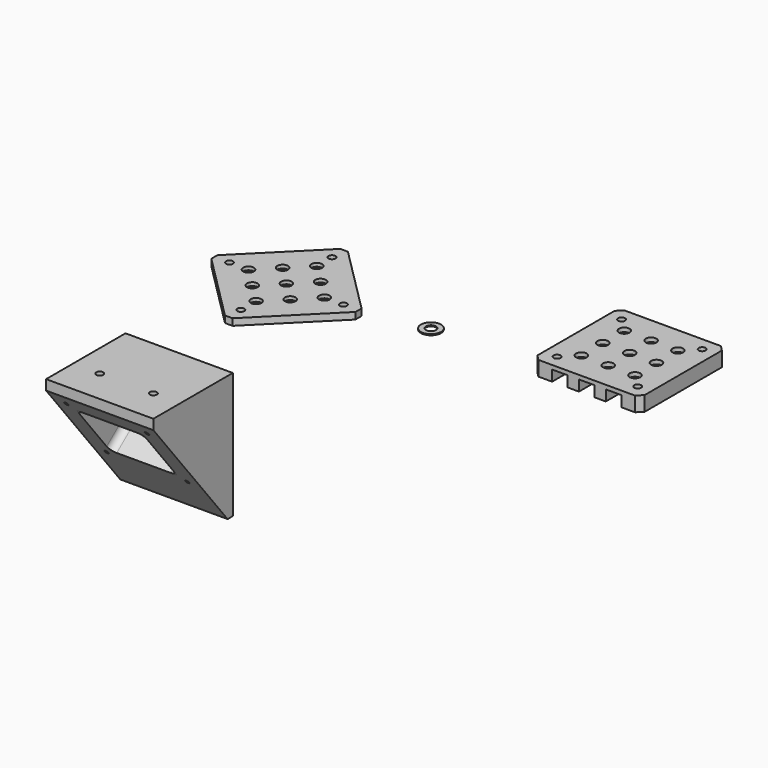
from build123d import *
from build123d import SkipClean  # not in build123d's __all__

# Parameters (mm, degrees)
F1_DEPTH        = 6.35
F2_D            = 6.604
F4_D            = 10.0838
F4_CBORE_D      = 19.558
F4_CBORE_DEPTH  = 3.175
F5_SIZE         = 5.08
F6_W            = 101.6
F6_H            = 101.6
F7_DEPTH        = 13.97
F9_D            = 6.604
F10_W           = 14.732
F10_H           = 10.16
F11_DEPTH       = 101.601
F12_SIZE        = 5.08
F13_R           = 9.525
F13_R_2         = 4.7625
F14_DEPTH       = 1.016
F16_DEPTH       = 50.8
F18_D           = 3.96875
F18_DEPTH       = 12.7
F18_TIP         = 1.1923327909
F20_DEPTH       = 119.0509465201
F22_D           = 6.604
F22_CBORE_D     = 10.16
F22_CBORE_DEPTH = 114.3
F23_W           = 63.5
F23_H           = 63.5
F24_DEPTH       = 31.75
F26_D           = 10.0838
F26_DEPTH       = 25.4
F26_TIP         = 3.0294791551
F27_T1_DEPTH    = 47.625
F27_T6_DEPTH    = 31.75
F27_S7_R        = 5.08
F27_T8_DEPTH    = 21
F27_T12_DEPTH   = 31.75
F27_S13_R       = 5.08
F27_T14_DEPTH   = 21


# Not quite as in the source:
# - a fillet or chamfer that OpenCascade refuses, or shapes differently, is made with other operations: its cross-section is extruded or revolved along the edge and cut away or added


with BuildPart() as f1:
    # F0 (on Top) → F1 (new body)
    with BuildSketch(Plane.XY):
        Polygon((-71.8420489686, 0), (0, -71.8420489686), (71.8420489686, 0), (0, 71.8420489686), align=None)
    extrude(amount=F1_DEPTH)

    # F2 (through all)
    with Locations(Plane(origin=(0, 0, 0), x_dir=(1, 0, 0), z_dir=(0, 0, -1))):
        with Locations((0, 53.975), (-53.975, 0), (53.975, 0), (0, -53.975)):
            Hole(F2_D / 2)

    # F4 (through all)
    with Locations(Plane(origin=(0, 0, 0), x_dir=(1, 0, 0), z_dir=(0, 0, -1))):
        with Locations((0, 35.9210244843), (-17.9605122421, 17.9605122421), (-35.9210244843, 0), (-17.9605122421, -17.9605122421), (0, -35.9210244843), (17.9605122421, -17.9605122421), (35.9210244843, 0), (17.9605122421, 17.9605122421), (0, 0)):
            CounterBoreHole(F4_D / 2, F4_CBORE_D / 2, F4_CBORE_DEPTH)

    # F5
    f5_edges = [f1.edges().sort_by_distance(p)[0] for p in [
        (-71.842049, 0, 3.175),
        (0, 71.842049, 3.175),
        (71.842049, 0, 3.175),
        (0, -71.842049, 3.175),
    ]]
    chamfer(f5_edges, length=F5_SIZE)


with BuildPart() as f7:
    # F6 (on face) → F7 (new body)
    with BuildSketch(Plane.XY.offset(6.35)):
        with Locations((284.3260511961, 50.8)):
            Rectangle(F6_W, F6_H)
    extrude(amount=F7_DEPTH)

    # F9 (through all)
    with Locations(Plane(origin=(0, 0, 6.35), x_dir=(1, 0, 0), z_dir=(0, 0, -1))):
        with Locations((246.1599626816, -88.9660885145), (246.1599626816, -12.6339114855), (322.4921397107, -12.6339114855), (322.4921397107, -88.9660885145)):
            Hole(F9_D / 2)

    # F10 (on face) → F11 (cut, through all)
    with BuildSketch(Plane.XZ):
        with Locations((309.7260511961, 11.43)):
            Rectangle(F10_W, F10_H)
        with Locations((284.3260511961, 11.43)):
            Rectangle(F10_W, F10_H)
        with Locations((258.9260511961, 11.43)):
            Rectangle(F10_W, F10_H)
    extrude(amount=-F11_DEPTH, mode=Mode.SUBTRACT)

    # F12
    f12_edges = [f7.edges().sort_by_distance(p)[0] for p in [
        (335.126051, 0, 13.335),
        (233.526051, 0, 13.335),
        (233.526051, 101.6, 13.335),
        (335.126051, 101.6, 13.335),
    ]]
    chamfer(f12_edges, length=F12_SIZE)

    # F26
    with Locations(Plane(origin=(0, 0, 16.51), x_dir=(1, 0, 0), z_dir=(0, 0, -1))):
        with Locations((258.9260511961, -25.4), (258.9260511961, -50.8), (258.9260511961, -76.2), (284.3260511961, -76.2), (284.3260511961, -50.8), (284.3260511961, -25.4), (309.7260511961, -25.4), (309.7260511961, -50.8), (309.7260511961, -76.2)):
            Hole(F26_D / 2, depth=F26_DEPTH)
            with Locations((0, 0, -(F26_DEPTH + F26_TIP / 2))):  # 118° drill point
                Cone(0, F26_D / 2, F26_TIP, mode=Mode.SUBTRACT)


with BuildPart() as f14:
    # F13 (on Top) → F14 (new body)
    with BuildSketch(Plane.XY):
        with Locations((121.6887831688, 18.9455170184)):
            Circle(F13_R)
        with Locations((121.6887831688, 18.9455170184)):
            Circle(F13_R_2, mode=Mode.SUBTRACT)
    extrude(amount=F14_DEPTH)


with BuildPart() as f16:
    # F15 (on Right) → F16 (new body, symmetric)
    with BuildSketch(Plane.YZ):
        Polygon((-127, 0), (-228.6, 0), (-127, -127), align=None)
    extrude(amount=F16_DEPTH, both=True)

    # F18
    with Locations(Plane(origin=(0, -139.3902439024, -111.512195122), x_dir=(1, 0, 0), z_dir=(0, -0.7808688094, -0.6246950476))):
        with Locations((38.1660885145, 41.1391993564), (-38.1660885145, 41.1391993564), (-38.1660885145, 117.4713763855), (38.1660885145, 117.4713763855)):
            Hole(F18_D / 2, depth=F18_DEPTH)
            with Locations((0, 0, -(F18_DEPTH + F18_TIP / 2))):  # 118° drill point
                Cone(0, F18_D / 2, F18_TIP, mode=Mode.SUBTRACT)

    # F19 (on face) → F20 (cut, through all)
    with BuildSketch(Plane.YZ.offset(50.8)):
        Polygon((-228.6, 0), (-220.98, -9.525), (-220.98, 0), align=None)
        Polygon((-127, -119.38), (-133.096, -119.38), (-127, -127), align=None)
    extrude(amount=-F20_DEPTH, mode=Mode.SUBTRACT)

    # F22 (through all)
    with Locations(Plane(origin=(0, 0, -119.38), x_dir=(1, 0, 0), z_dir=(0, 0, -1))):
        with Locations((-25.4, 189.23), (25.4, 189.23)):
            CounterBoreHole(F22_D / 2, F22_CBORE_D / 2, F22_CBORE_DEPTH)

    # F23 (on face) → F24 (cut)
    with BuildSketch(Plane(origin=(0, -139.3902439024, -111.512195122), x_dir=(1, 0, 0), z_dir=(0, -0.7808688094, -0.6246950476))):
        with Locations((0, 79.3052878709)):
            Rectangle(F23_W, F23_H)
    extrude(amount=-F24_DEPTH, mode=Mode.SUBTRACT)

    # F27: fillet of radius 6.35 on 4 edges, made by hand

    # F27_s2 → F27_t1 (join)
    with BuildSketch(Plane(origin=(0, -139.3902439024, -111.512195122), x_dir=(1, 0, 0), z_dir=(0, 0.7808688094, 0.6246950476))):
        with BuildLine():
            ThreePointArc((-31.75, -53.9052878709), (-29.8901280605, -49.4151598104), (-25.4, -47.5552878709))
            Line((-25.4, -47.5552878709), (-31.75, -47.5552878709))
            Line((-31.75, -47.5552878709), (-31.75, -53.9052878709))
        make_face()
        with BuildLine():
            ThreePointArc((25.4, -47.5552878709), (29.8901280605, -49.4151598104), (31.75, -53.9052878709))
            Line((31.75, -53.9052878709), (31.75, -47.5552878709))
            Line((31.75, -47.5552878709), (25.4, -47.5552878709))
        make_face()
    extrude(amount=F27_T1_DEPTH)


with BuildPart() as f27_tool4:
    # F27_s5 → F27_t6 (new body)
    with BuildSketch(Plane(origin=(0, -139.3902439024, -111.512195122), x_dir=(1, 0, 0), z_dir=(0, 0.7808688094, 0.6246950476))):
        with BuildLine():
            ThreePointArc((-31.75, -104.7052878709), (-29.8901280605, -109.1954159315), (-25.4, -111.0552878709))
            Line((-25.4, -111.0552878709), (-31.75, -111.0552878709))
            Line((-31.75, -111.0552878709), (-31.75, -104.7052878709))
        make_face()
    extrude(amount=F27_T6_DEPTH)

    # F27_s7 → F27_t8 (cut, symmetric)
    with BuildSketch(Plane.XY.offset(-17.4)):
        with Locations((-25.4, -189.23)):
            Circle(F27_S7_R)
    extrude(amount=F27_T8_DEPTH, both=True, mode=Mode.SUBTRACT)


with BuildPart() as f16_1:
    add(f16.part, clean=False)

    # F27_t3: union F27_tool4
    add(f27_tool4.part)


with BuildPart() as f27_tool10:
    # F27_s11 → F27_t12 (new body)
    with BuildSketch(Plane(origin=(0, -139.3902439024, -111.512195122), x_dir=(1, 0, 0), z_dir=(0, 0.7808688094, 0.6246950476))):
        with BuildLine():
            ThreePointArc((31.75, -104.7052878709), (29.8901280605, -109.1954159315), (25.4, -111.0552878709))
            Line((25.4, -111.0552878709), (31.75, -111.0552878709))
            Line((31.75, -111.0552878709), (31.75, -104.7052878709))
        make_face()
    extrude(amount=F27_T12_DEPTH)

    # F27_s13 → F27_t14 (cut, symmetric)
    with BuildSketch(Plane.XY.offset(-17.4)):
        with Locations((25.4, -189.23)):
            Circle(F27_S13_R)
    with SkipClean():  # cleaning this boolean's faces spoils the solid; the shape is the same uncleaned
        extrude(amount=F27_T14_DEPTH, both=True, mode=Mode.SUBTRACT)


with BuildPart() as f16_2:
    add(f16_1.part, clean=False)

    # F27_t9: union F27_tool10
    add(f27_tool10.part)


solid = Compound([f1.part, f7.part, f14.part, f16_2.part])
